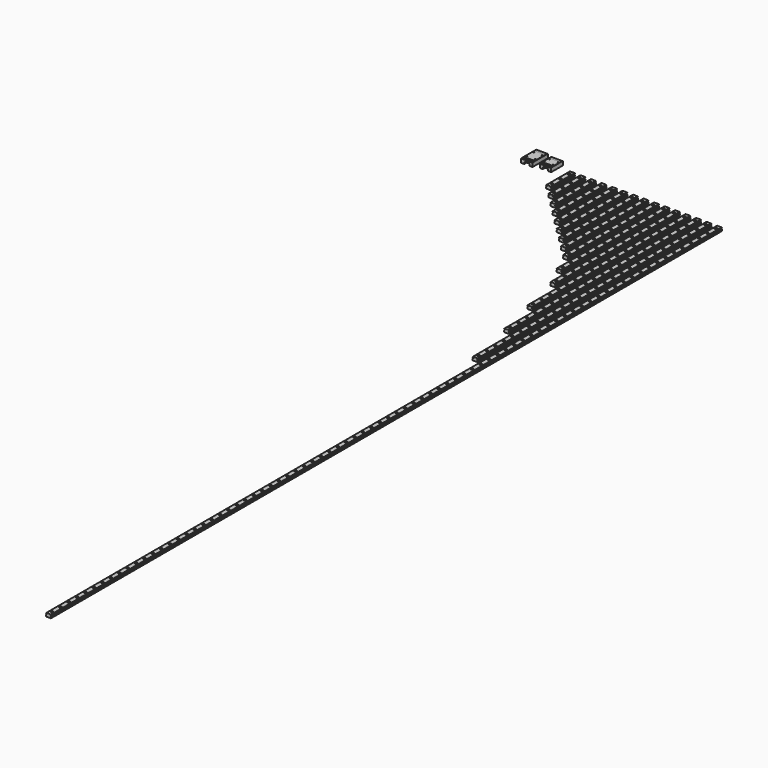
from build123d import *

# Parameters (mm, degrees)
F1_DEPTH           = 70
F2_DEPTH           = 95
F3_DEPTH           = 120
F4_DEPTH           = 145
F5_DEPTH           = 170
F6_DEPTH           = 195
F7_DEPTH           = 220
F8_DEPTH           = 245
F9_DEPTH           = 270
F10_DEPTH          = 320
F11_DEPTH          = 370
F12_DEPTH          = 470
F13_DEPTH          = 570
F14_DEPTH          = 695
F15_DEPTH          = 1995
F17_D              = 3.5
F17_CBORE_D        = 6
F17_CBORE_DEPTH    = 4.5
F17_2_D            = 3.5
F17_2_CBORE_D      = 6
F17_2_CBORE_DEPTH  = 4.5
F17_3_D            = 3.5
F17_3_CBORE_D      = 6
F17_3_CBORE_DEPTH  = 4.5
F17_4_D            = 3.5
F17_4_CBORE_D      = 6
F17_4_CBORE_DEPTH  = 4.5
F17_5_D            = 3.5
F17_5_CBORE_D      = 6
F17_5_CBORE_DEPTH  = 4.5
F17_6_D            = 3.5
F17_6_CBORE_D      = 6
F17_6_CBORE_DEPTH  = 4.5
F17_7_D            = 3.5
F17_7_CBORE_D      = 6
F17_7_CBORE_DEPTH  = 4.5
F17_8_D            = 3.5
F17_8_CBORE_D      = 6
F17_8_CBORE_DEPTH  = 4.5
F17_9_D            = 3.5
F17_9_CBORE_D      = 6
F17_9_CBORE_DEPTH  = 4.5
F17_10_D           = 3.5
F17_10_CBORE_D     = 6
F17_10_CBORE_DEPTH = 4.5
F18_D              = 3.5
F18_CBORE_D        = 6
F18_CBORE_DEPTH    = 4.5
F18_2_D            = 3.5
F18_2_CBORE_D      = 6
F18_2_CBORE_DEPTH  = 4.5
F18_3_D            = 3.5
F18_3_CBORE_D      = 6
F18_3_CBORE_DEPTH  = 4.5
F18_4_D            = 3.5
F18_4_CBORE_D      = 6
F18_4_CBORE_DEPTH  = 4.5
F19_D              = 3.5
F19_CBORE_D        = 6
F19_CBORE_DEPTH    = 4.5
F21_DEPTH          = 10.85
F23_DEPTH          = 6.5
F24_DEPTH          = 16.2
F26_DEPTH          = 6.5
F28_D              = 2.5
F28_DEPTH          = 5
F28_TIP            = 0.7510757738
F28_2_D            = 2.5
F28_2_DEPTH        = 5
F28_2_TIP          = 0.7510757738
F29_SIZE           = 0.49999
F29_2_SIZE         = 0.49999


# Not quite as in the source:
# - a fillet or chamfer is up to 0.001 mm smaller than in the source, because OpenCascade refuses the exact size


with BuildPart() as f1:
    # F0 (on Front) → F1 (new body)
    with BuildSketch(Plane.XZ):
        with BuildLine():
            Line((-5.5050252532, -4), (5.5050252532, -4))
            Line((5.5050252532, -4), (6, -3.5050252532))
            Line((6, -3.5050252532), (6, -0.0298848634))
            ThreePointArc((6, -0.0298848634), (5.4909752969, 0.2684521405), (5.150060681, 0.75))
            Line((5.150060681, 0.75), (4.45, 0.75))
            Line((4.45, 0.75), (4.45, 1.85))
            Line((4.45, 1.85), (5.150060681, 1.85))
            ThreePointArc((5.150060681, 1.85), (5.4909752969, 2.3315478595), (6, 2.6298848634))
            Line((6, 2.6298848634), (6, 3.5050252532))
            Line((6, 3.5050252532), (5.5050252532, 4))
            Line((5.5050252532, 4), (-5.5050252532, 4))
            Line((-5.5050252532, 4), (-6, 3.5050252532))
            Line((-6, 3.5050252532), (-6, 2.6298848634))
            ThreePointArc((-6, 2.6298848634), (-5.4909752969, 2.3315478595), (-5.150060681, 1.85))
            Line((-5.150060681, 1.85), (-4.45, 1.85))
            Line((-4.45, 1.85), (-4.45, 0.75))
            Line((-4.45, 0.75), (-5.150060681, 0.75))
            ThreePointArc((-5.150060681, 0.75), (-5.4909752969, 0.2684521405), (-6, -0.0298848634))
            Line((-6, -0.0298848634), (-6, -3.5050252532))
            Line((-6, -3.5050252532), (-5.5050252532, -4))
        make_face()
    extrude(amount=F1_DEPTH)

    # F17 (through all)
    with Locations(Plane.XY.offset(4)):
        with Locations((150, -10), (225, -35), (225, -10), (225, -60), (50, -60), (25, -10), (125, -60), (200, -10), (75, -10), (175, -35), (25, -60), (0, -35), (175, -10), (200, -35), (200, -60), (75, -60), (150, -60), (50, -35), (100, -10), (150, -35), (25, -35), (175, -60), (0, -10), (125, -35), (50, -10), (125, -10), (100, -35), (75, -35), (0, -60), (100, -60), (150, -85), (100, -85), (225, -85), (175, -85), (75, -85), (125, -85), (25, -85), (200, -85), (50, -85), (50, -110), (225, -110), (225, -135), (200, -110), (125, -110), (75, -110), (100, -135), (150, -135), (125, -135), (175, -135), (100, -110), (200, -135), (75, -135), (175, -110), (150, -110), (200, -160), (150, -160), (125, -160), (175, -160), (100, -160), (225, -160), (175, -185), (200, -185), (150, -185), (125, -185), (225, -185), (200, -260), (225, -310), (225, -260), (225, -285), (150, -210), (200, -235), (225, -210), (225, -235), (200, -210), (175, -235), (175, -210)):
            CounterBoreHole(F17_D / 2, F17_CBORE_D / 2, F17_CBORE_DEPTH)


with BuildPart() as f2:
    # F0 (on Front) → F2 (new body)
    with BuildSketch(Plane.XZ):
        with BuildLine():
            Line((19, -0.0298848634), (19, -3.5050252532))
            Line((19, -3.5050252532), (19.4949747468, -4))
            Line((19.4949747468, -4), (30.5050252532, -4))
            Line((30.5050252532, -4), (31, -3.5050252532))
            Line((31, -3.5050252532), (31, -0.0298848634))
            ThreePointArc((31, -0.0298848634), (30.4909752969, 0.2684521405), (30.150060681, 0.75))
            Line((30.150060681, 0.75), (29.45, 0.75))
            Line((29.45, 0.75), (29.45, 1.85))
            Line((29.45, 1.85), (30.150060681, 1.85))
            ThreePointArc((30.150060681, 1.85), (30.4909752969, 2.3315478595), (31, 2.6298848634))
            Line((31, 2.6298848634), (31, 3.5050252532))
            Line((31, 3.5050252532), (30.5050252532, 4))
            Line((30.5050252532, 4), (19.4949747468, 4))
            Line((19.4949747468, 4), (19, 3.5050252532))
            Line((19, 3.5050252532), (19, 2.6298848634))
            ThreePointArc((19, 2.6298848634), (19.5090247031, 2.3315478595), (19.849939319, 1.85))
            Line((19.849939319, 1.85), (20.55, 1.85))
            Line((20.55, 1.85), (20.55, 0.75))
            Line((20.55, 0.75), (19.849939319, 0.75))
            ThreePointArc((19.849939319, 0.75), (19.5090247031, 0.2684521405), (19, -0.0298848634))
        make_face()
    extrude(amount=F2_DEPTH)

    # F17#2 (through all)
    with Locations(Plane.XY.offset(4)):
        with Locations((150, -10), (225, -35), (225, -10), (225, -60), (50, -60), (25, -10), (125, -60), (200, -10), (75, -10), (175, -35), (25, -60), (0, -35), (175, -10), (200, -35), (200, -60), (75, -60), (150, -60), (50, -35), (100, -10), (150, -35), (25, -35), (175, -60), (0, -10), (125, -35), (50, -10), (125, -10), (100, -35), (75, -35), (0, -60), (100, -60), (150, -85), (100, -85), (225, -85), (175, -85), (75, -85), (125, -85), (25, -85), (200, -85), (50, -85), (50, -110), (225, -110), (225, -135), (200, -110), (125, -110), (75, -110), (100, -135), (150, -135), (125, -135), (175, -135), (100, -110), (200, -135), (75, -135), (175, -110), (150, -110), (200, -160), (150, -160), (125, -160), (175, -160), (100, -160), (225, -160), (175, -185), (200, -185), (150, -185), (125, -185), (225, -185), (200, -260), (225, -310), (225, -260), (225, -285), (150, -210), (200, -235), (225, -210), (225, -235), (200, -210), (175, -235), (175, -210)):
            CounterBoreHole(F17_2_D / 2, F17_2_CBORE_D / 2, F17_2_CBORE_DEPTH)


with BuildPart() as f3:
    # F0 (on Front) → F3 (new body)
    with BuildSketch(Plane.XZ):
        with BuildLine():
            Line((44, -0.0298848634), (44, -3.5050252532))
            Line((44, -3.5050252532), (44.4949747468, -4))
            Line((44.4949747468, -4), (55.5050252532, -4))
            Line((55.5050252532, -4), (56, -3.5050252532))
            Line((56, -3.5050252532), (56, -0.0298848634))
            ThreePointArc((56, -0.0298848634), (55.4909752969, 0.2684521405), (55.150060681, 0.75))
            Line((55.150060681, 0.75), (54.45, 0.75))
            Line((54.45, 0.75), (54.45, 1.85))
            Line((54.45, 1.85), (55.150060681, 1.85))
            ThreePointArc((55.150060681, 1.85), (55.4909752969, 2.3315478595), (56, 2.6298848634))
            Line((56, 2.6298848634), (56, 3.5050252532))
            Line((56, 3.5050252532), (55.5050252532, 4))
            Line((55.5050252532, 4), (44.4949747468, 4))
            Line((44.4949747468, 4), (44, 3.5050252532))
            Line((44, 3.5050252532), (44, 2.6298848634))
            ThreePointArc((44, 2.6298848634), (44.5090247031, 2.3315478595), (44.849939319, 1.85))
            Line((44.849939319, 1.85), (45.55, 1.85))
            Line((45.55, 1.85), (45.55, 0.75))
            Line((45.55, 0.75), (44.849939319, 0.75))
            ThreePointArc((44.849939319, 0.75), (44.5090247031, 0.2684521405), (44, -0.0298848634))
        make_face()
    extrude(amount=F3_DEPTH)

    # F17#3 (through all)
    with Locations(Plane.XY.offset(4)):
        with Locations((150, -10), (225, -35), (225, -10), (225, -60), (50, -60), (25, -10), (125, -60), (200, -10), (75, -10), (175, -35), (25, -60), (0, -35), (175, -10), (200, -35), (200, -60), (75, -60), (150, -60), (50, -35), (100, -10), (150, -35), (25, -35), (175, -60), (0, -10), (125, -35), (50, -10), (125, -10), (100, -35), (75, -35), (0, -60), (100, -60), (150, -85), (100, -85), (225, -85), (175, -85), (75, -85), (125, -85), (25, -85), (200, -85), (50, -85), (50, -110), (225, -110), (225, -135), (200, -110), (125, -110), (75, -110), (100, -135), (150, -135), (125, -135), (175, -135), (100, -110), (200, -135), (75, -135), (175, -110), (150, -110), (200, -160), (150, -160), (125, -160), (175, -160), (100, -160), (225, -160), (175, -185), (200, -185), (150, -185), (125, -185), (225, -185), (200, -260), (225, -310), (225, -260), (225, -285), (150, -210), (200, -235), (225, -210), (225, -235), (200, -210), (175, -235), (175, -210)):
            CounterBoreHole(F17_3_D / 2, F17_3_CBORE_D / 2, F17_3_CBORE_DEPTH)


with BuildPart() as f4:
    # F0 (on Front) → F4 (new body)
    with BuildSketch(Plane.XZ):
        with BuildLine():
            Line((69, -0.0298848634), (69, -3.5050252532))
            Line((69, -3.5050252532), (69.4949747468, -4))
            Line((69.4949747468, -4), (80.5050252532, -4))
            Line((80.5050252532, -4), (81, -3.5050252532))
            Line((81, -3.5050252532), (81, -0.0298848634))
            ThreePointArc((81, -0.0298848634), (80.4909752969, 0.2684521405), (80.150060681, 0.75))
            Line((80.150060681, 0.75), (79.45, 0.75))
            Line((79.45, 0.75), (79.45, 1.85))
            Line((79.45, 1.85), (80.150060681, 1.85))
            ThreePointArc((80.150060681, 1.85), (80.4909752969, 2.3315478595), (81, 2.6298848634))
            Line((81, 2.6298848634), (81, 3.5050252532))
            Line((81, 3.5050252532), (80.5050252532, 4))
            Line((80.5050252532, 4), (69.4949747468, 4))
            Line((69.4949747468, 4), (69, 3.5050252532))
            Line((69, 3.5050252532), (69, 2.6298848634))
            ThreePointArc((69, 2.6298848634), (69.5090247031, 2.3315478595), (69.849939319, 1.85))
            Line((69.849939319, 1.85), (70.55, 1.85))
            Line((70.55, 1.85), (70.55, 0.75))
            Line((70.55, 0.75), (69.849939319, 0.75))
            ThreePointArc((69.849939319, 0.75), (69.5090247031, 0.2684521405), (69, -0.0298848634))
        make_face()
    extrude(amount=F4_DEPTH)

    # F17#4 (through all)
    with Locations(Plane.XY.offset(4)):
        with Locations((150, -10), (225, -35), (225, -10), (225, -60), (50, -60), (25, -10), (125, -60), (200, -10), (75, -10), (175, -35), (25, -60), (0, -35), (175, -10), (200, -35), (200, -60), (75, -60), (150, -60), (50, -35), (100, -10), (150, -35), (25, -35), (175, -60), (0, -10), (125, -35), (50, -10), (125, -10), (100, -35), (75, -35), (0, -60), (100, -60), (150, -85), (100, -85), (225, -85), (175, -85), (75, -85), (125, -85), (25, -85), (200, -85), (50, -85), (50, -110), (225, -110), (225, -135), (200, -110), (125, -110), (75, -110), (100, -135), (150, -135), (125, -135), (175, -135), (100, -110), (200, -135), (75, -135), (175, -110), (150, -110), (200, -160), (150, -160), (125, -160), (175, -160), (100, -160), (225, -160), (175, -185), (200, -185), (150, -185), (125, -185), (225, -185), (200, -260), (225, -310), (225, -260), (225, -285), (150, -210), (200, -235), (225, -210), (225, -235), (200, -210), (175, -235), (175, -210)):
            CounterBoreHole(F17_4_D / 2, F17_4_CBORE_D / 2, F17_4_CBORE_DEPTH)


with BuildPart() as f5:
    # F0 (on Front) → F5 (new body)
    with BuildSketch(Plane.XZ):
        with BuildLine():
            Line((94, -0.0298848634), (94, -3.5050252532))
            Line((94, -3.5050252532), (94.4949747468, -4))
            Line((94.4949747468, -4), (105.5050252532, -4))
            Line((105.5050252532, -4), (106, -3.5050252532))
            Line((106, -3.5050252532), (106, -0.0298848634))
            ThreePointArc((106, -0.0298848634), (105.4909752969, 0.2684521405), (105.150060681, 0.75))
            Line((105.150060681, 0.75), (104.45, 0.75))
            Line((104.45, 0.75), (104.45, 1.85))
            Line((104.45, 1.85), (105.150060681, 1.85))
            ThreePointArc((105.150060681, 1.85), (105.4909752969, 2.3315478595), (106, 2.6298848634))
            Line((106, 2.6298848634), (106, 3.5050252532))
            Line((106, 3.5050252532), (105.5050252532, 4))
            Line((105.5050252532, 4), (94.4949747468, 4))
            Line((94.4949747468, 4), (94, 3.5050252532))
            Line((94, 3.5050252532), (94, 2.6298848634))
            ThreePointArc((94, 2.6298848634), (94.5090247031, 2.3315478595), (94.849939319, 1.85))
            Line((94.849939319, 1.85), (95.55, 1.85))
            Line((95.55, 1.85), (95.55, 0.75))
            Line((95.55, 0.75), (94.849939319, 0.75))
            ThreePointArc((94.849939319, 0.75), (94.5090247031, 0.2684521405), (94, -0.0298848634))
        make_face()
    extrude(amount=F5_DEPTH)

    # F17#5 (through all)
    with Locations(Plane.XY.offset(4)):
        with Locations((150, -10), (225, -35), (225, -10), (225, -60), (50, -60), (25, -10), (125, -60), (200, -10), (75, -10), (175, -35), (25, -60), (0, -35), (175, -10), (200, -35), (200, -60), (75, -60), (150, -60), (50, -35), (100, -10), (150, -35), (25, -35), (175, -60), (0, -10), (125, -35), (50, -10), (125, -10), (100, -35), (75, -35), (0, -60), (100, -60), (150, -85), (100, -85), (225, -85), (175, -85), (75, -85), (125, -85), (25, -85), (200, -85), (50, -85), (50, -110), (225, -110), (225, -135), (200, -110), (125, -110), (75, -110), (100, -135), (150, -135), (125, -135), (175, -135), (100, -110), (200, -135), (75, -135), (175, -110), (150, -110), (200, -160), (150, -160), (125, -160), (175, -160), (100, -160), (225, -160), (175, -185), (200, -185), (150, -185), (125, -185), (225, -185), (200, -260), (225, -310), (225, -260), (225, -285), (150, -210), (200, -235), (225, -210), (225, -235), (200, -210), (175, -235), (175, -210)):
            CounterBoreHole(F17_5_D / 2, F17_5_CBORE_D / 2, F17_5_CBORE_DEPTH)


with BuildPart() as f6:
    # F0 (on Front) → F6 (new body)
    with BuildSketch(Plane.XZ):
        with BuildLine():
            Line((119, -0.0298848634), (119, -3.5050252532))
            Line((119, -3.5050252532), (119.4949747468, -4))
            Line((119.4949747468, -4), (130.5050252532, -4))
            Line((130.5050252532, -4), (131, -3.5050252532))
            Line((131, -3.5050252532), (131, -0.0298848634))
            ThreePointArc((131, -0.0298848634), (130.4909752969, 0.2684521405), (130.150060681, 0.75))
            Line((130.150060681, 0.75), (129.45, 0.75))
            Line((129.45, 0.75), (129.45, 1.85))
            Line((129.45, 1.85), (130.150060681, 1.85))
            ThreePointArc((130.150060681, 1.85), (130.4909752969, 2.3315478595), (131, 2.6298848634))
            Line((131, 2.6298848634), (131, 3.5050252532))
            Line((131, 3.5050252532), (130.5050252532, 4))
            Line((130.5050252532, 4), (119.4949747468, 4))
            Line((119.4949747468, 4), (119, 3.5050252532))
            Line((119, 3.5050252532), (119, 2.6298848634))
            ThreePointArc((119, 2.6298848634), (119.5090247031, 2.3315478595), (119.849939319, 1.85))
            Line((119.849939319, 1.85), (120.55, 1.85))
            Line((120.55, 1.85), (120.55, 0.75))
            Line((120.55, 0.75), (119.849939319, 0.75))
            ThreePointArc((119.849939319, 0.75), (119.5090247031, 0.2684521405), (119, -0.0298848634))
        make_face()
    extrude(amount=F6_DEPTH)

    # F17#6 (through all)
    with Locations(Plane.XY.offset(4)):
        with Locations((150, -10), (225, -35), (225, -10), (225, -60), (50, -60), (25, -10), (125, -60), (200, -10), (75, -10), (175, -35), (25, -60), (0, -35), (175, -10), (200, -35), (200, -60), (75, -60), (150, -60), (50, -35), (100, -10), (150, -35), (25, -35), (175, -60), (0, -10), (125, -35), (50, -10), (125, -10), (100, -35), (75, -35), (0, -60), (100, -60), (150, -85), (100, -85), (225, -85), (175, -85), (75, -85), (125, -85), (25, -85), (200, -85), (50, -85), (50, -110), (225, -110), (225, -135), (200, -110), (125, -110), (75, -110), (100, -135), (150, -135), (125, -135), (175, -135), (100, -110), (200, -135), (75, -135), (175, -110), (150, -110), (200, -160), (150, -160), (125, -160), (175, -160), (100, -160), (225, -160), (175, -185), (200, -185), (150, -185), (125, -185), (225, -185), (200, -260), (225, -310), (225, -260), (225, -285), (150, -210), (200, -235), (225, -210), (225, -235), (200, -210), (175, -235), (175, -210)):
            CounterBoreHole(F17_6_D / 2, F17_6_CBORE_D / 2, F17_6_CBORE_DEPTH)


with BuildPart() as f7:
    # F0 (on Front) → F7 (new body)
    with BuildSketch(Plane.XZ):
        with BuildLine():
            Line((144, -0.0298848634), (144, -3.5050252532))
            Line((144, -3.5050252532), (144.4949747468, -4))
            Line((144.4949747468, -4), (155.5050252532, -4))
            Line((155.5050252532, -4), (156, -3.5050252532))
            Line((156, -3.5050252532), (156, -0.0298848634))
            ThreePointArc((156, -0.0298848634), (155.4909752969, 0.2684521405), (155.150060681, 0.75))
            Line((155.150060681, 0.75), (154.45, 0.75))
            Line((154.45, 0.75), (154.45, 1.85))
            Line((154.45, 1.85), (155.150060681, 1.85))
            ThreePointArc((155.150060681, 1.85), (155.4909752969, 2.3315478595), (156, 2.6298848634))
            Line((156, 2.6298848634), (156, 3.5050252532))
            Line((156, 3.5050252532), (155.5050252532, 4))
            Line((155.5050252532, 4), (144.4949747468, 4))
            Line((144.4949747468, 4), (144, 3.5050252532))
            Line((144, 3.5050252532), (144, 2.6298848634))
            ThreePointArc((144, 2.6298848634), (144.5090247031, 2.3315478595), (144.849939319, 1.85))
            Line((144.849939319, 1.85), (145.55, 1.85))
            Line((145.55, 1.85), (145.55, 0.75))
            Line((145.55, 0.75), (144.849939319, 0.75))
            ThreePointArc((144.849939319, 0.75), (144.5090247031, 0.2684521405), (144, -0.0298848634))
        make_face()
    extrude(amount=F7_DEPTH)

    # F17#7 (through all)
    with Locations(Plane.XY.offset(4)):
        with Locations((150, -10), (225, -35), (225, -10), (225, -60), (50, -60), (25, -10), (125, -60), (200, -10), (75, -10), (175, -35), (25, -60), (0, -35), (175, -10), (200, -35), (200, -60), (75, -60), (150, -60), (50, -35), (100, -10), (150, -35), (25, -35), (175, -60), (0, -10), (125, -35), (50, -10), (125, -10), (100, -35), (75, -35), (0, -60), (100, -60), (150, -85), (100, -85), (225, -85), (175, -85), (75, -85), (125, -85), (25, -85), (200, -85), (50, -85), (50, -110), (225, -110), (225, -135), (200, -110), (125, -110), (75, -110), (100, -135), (150, -135), (125, -135), (175, -135), (100, -110), (200, -135), (75, -135), (175, -110), (150, -110), (200, -160), (150, -160), (125, -160), (175, -160), (100, -160), (225, -160), (175, -185), (200, -185), (150, -185), (125, -185), (225, -185), (200, -260), (225, -310), (225, -260), (225, -285), (150, -210), (200, -235), (225, -210), (225, -235), (200, -210), (175, -235), (175, -210)):
            CounterBoreHole(F17_7_D / 2, F17_7_CBORE_D / 2, F17_7_CBORE_DEPTH)


with BuildPart() as f8:
    # F0 (on Front) → F8 (new body)
    with BuildSketch(Plane.XZ):
        with BuildLine():
            Line((169, -0.0298848634), (169, -3.5050252532))
            Line((169, -3.5050252532), (169.4949747468, -4))
            Line((169.4949747468, -4), (180.5050252532, -4))
            Line((180.5050252532, -4), (181, -3.5050252532))
            Line((181, -3.5050252532), (181, -0.0298848634))
            ThreePointArc((181, -0.0298848634), (180.4909752969, 0.2684521405), (180.150060681, 0.75))
            Line((180.150060681, 0.75), (179.45, 0.75))
            Line((179.45, 0.75), (179.45, 1.85))
            Line((179.45, 1.85), (180.150060681, 1.85))
            ThreePointArc((180.150060681, 1.85), (180.4909752969, 2.3315478595), (181, 2.6298848634))
            Line((181, 2.6298848634), (181, 3.5050252532))
            Line((181, 3.5050252532), (180.5050252532, 4))
            Line((180.5050252532, 4), (169.4949747468, 4))
            Line((169.4949747468, 4), (169, 3.5050252532))
            Line((169, 3.5050252532), (169, 2.6298848634))
            ThreePointArc((169, 2.6298848634), (169.5090247031, 2.3315478595), (169.849939319, 1.85))
            Line((169.849939319, 1.85), (170.55, 1.85))
            Line((170.55, 1.85), (170.55, 0.75))
            Line((170.55, 0.75), (169.849939319, 0.75))
            ThreePointArc((169.849939319, 0.75), (169.5090247031, 0.2684521405), (169, -0.0298848634))
        make_face()
    extrude(amount=F8_DEPTH)

    # F17#8 (through all)
    with Locations(Plane.XY.offset(4)):
        with Locations((150, -10), (225, -35), (225, -10), (225, -60), (50, -60), (25, -10), (125, -60), (200, -10), (75, -10), (175, -35), (25, -60), (0, -35), (175, -10), (200, -35), (200, -60), (75, -60), (150, -60), (50, -35), (100, -10), (150, -35), (25, -35), (175, -60), (0, -10), (125, -35), (50, -10), (125, -10), (100, -35), (75, -35), (0, -60), (100, -60), (150, -85), (100, -85), (225, -85), (175, -85), (75, -85), (125, -85), (25, -85), (200, -85), (50, -85), (50, -110), (225, -110), (225, -135), (200, -110), (125, -110), (75, -110), (100, -135), (150, -135), (125, -135), (175, -135), (100, -110), (200, -135), (75, -135), (175, -110), (150, -110), (200, -160), (150, -160), (125, -160), (175, -160), (100, -160), (225, -160), (175, -185), (200, -185), (150, -185), (125, -185), (225, -185), (200, -260), (225, -310), (225, -260), (225, -285), (150, -210), (200, -235), (225, -210), (225, -235), (200, -210), (175, -235), (175, -210)):
            CounterBoreHole(F17_8_D / 2, F17_8_CBORE_D / 2, F17_8_CBORE_DEPTH)


with BuildPart() as f9:
    # F0 (on Front) → F9 (new body)
    with BuildSketch(Plane.XZ):
        with BuildLine():
            Line((194, -0.0298848634), (194, -3.5050252532))
            Line((194, -3.5050252532), (194.4949747468, -4))
            Line((194.4949747468, -4), (205.5050252532, -4))
            Line((205.5050252532, -4), (206, -3.5050252532))
            Line((206, -3.5050252532), (206, -0.0298848634))
            ThreePointArc((206, -0.0298848634), (205.4909752969, 0.2684521405), (205.150060681, 0.75))
            Line((205.150060681, 0.75), (204.45, 0.75))
            Line((204.45, 0.75), (204.45, 1.85))
            Line((204.45, 1.85), (205.150060681, 1.85))
            ThreePointArc((205.150060681, 1.85), (205.4909752969, 2.3315478595), (206, 2.6298848634))
            Line((206, 2.6298848634), (206, 3.5050252532))
            Line((206, 3.5050252532), (205.5050252532, 4))
            Line((205.5050252532, 4), (194.4949747468, 4))
            Line((194.4949747468, 4), (194, 3.5050252532))
            Line((194, 3.5050252532), (194, 2.6298848634))
            ThreePointArc((194, 2.6298848634), (194.5090247031, 2.3315478595), (194.849939319, 1.85))
            Line((194.849939319, 1.85), (195.55, 1.85))
            Line((195.55, 1.85), (195.55, 0.75))
            Line((195.55, 0.75), (194.849939319, 0.75))
            ThreePointArc((194.849939319, 0.75), (194.5090247031, 0.2684521405), (194, -0.0298848634))
        make_face()
    extrude(amount=F9_DEPTH)

    # F17#9 (through all)
    with Locations(Plane.XY.offset(4)):
        with Locations((150, -10), (225, -35), (225, -10), (225, -60), (50, -60), (25, -10), (125, -60), (200, -10), (75, -10), (175, -35), (25, -60), (0, -35), (175, -10), (200, -35), (200, -60), (75, -60), (150, -60), (50, -35), (100, -10), (150, -35), (25, -35), (175, -60), (0, -10), (125, -35), (50, -10), (125, -10), (100, -35), (75, -35), (0, -60), (100, -60), (150, -85), (100, -85), (225, -85), (175, -85), (75, -85), (125, -85), (25, -85), (200, -85), (50, -85), (50, -110), (225, -110), (225, -135), (200, -110), (125, -110), (75, -110), (100, -135), (150, -135), (125, -135), (175, -135), (100, -110), (200, -135), (75, -135), (175, -110), (150, -110), (200, -160), (150, -160), (125, -160), (175, -160), (100, -160), (225, -160), (175, -185), (200, -185), (150, -185), (125, -185), (225, -185), (200, -260), (225, -310), (225, -260), (225, -285), (150, -210), (200, -235), (225, -210), (225, -235), (200, -210), (175, -235), (175, -210)):
            CounterBoreHole(F17_9_D / 2, F17_9_CBORE_D / 2, F17_9_CBORE_DEPTH)


with BuildPart() as f10:
    # F0 (on Front) → F10 (new body)
    with BuildSketch(Plane.XZ):
        with BuildLine():
            Line((219, -0.0298848634), (219, -3.5050252532))
            Line((219, -3.5050252532), (219.4949747468, -4))
            Line((219.4949747468, -4), (230.5050252532, -4))
            Line((230.5050252532, -4), (231, -3.5050252532))
            Line((231, -3.5050252532), (231, -0.0298848634))
            ThreePointArc((231, -0.0298848634), (230.4909752969, 0.2684521405), (230.150060681, 0.75))
            Line((230.150060681, 0.75), (229.45, 0.75))
            Line((229.45, 0.75), (229.45, 1.85))
            Line((229.45, 1.85), (230.150060681, 1.85))
            ThreePointArc((230.150060681, 1.85), (230.4909752969, 2.3315478595), (231, 2.6298848634))
            Line((231, 2.6298848634), (231, 3.5050252532))
            Line((231, 3.5050252532), (230.5050252532, 4))
            Line((230.5050252532, 4), (219.4949747468, 4))
            Line((219.4949747468, 4), (219, 3.5050252532))
            Line((219, 3.5050252532), (219, 2.6298848634))
            ThreePointArc((219, 2.6298848634), (219.5090247031, 2.3315478595), (219.849939319, 1.85))
            Line((219.849939319, 1.85), (220.55, 1.85))
            Line((220.55, 1.85), (220.55, 0.75))
            Line((220.55, 0.75), (219.849939319, 0.75))
            ThreePointArc((219.849939319, 0.75), (219.5090247031, 0.2684521405), (219, -0.0298848634))
        make_face()
    extrude(amount=F10_DEPTH)

    # F17#10 (through all)
    with Locations(Plane.XY.offset(4)):
        with Locations((150, -10), (225, -35), (225, -10), (225, -60), (50, -60), (25, -10), (125, -60), (200, -10), (75, -10), (175, -35), (25, -60), (0, -35), (175, -10), (200, -35), (200, -60), (75, -60), (150, -60), (50, -35), (100, -10), (150, -35), (25, -35), (175, -60), (0, -10), (125, -35), (50, -10), (125, -10), (100, -35), (75, -35), (0, -60), (100, -60), (150, -85), (100, -85), (225, -85), (175, -85), (75, -85), (125, -85), (25, -85), (200, -85), (50, -85), (50, -110), (225, -110), (225, -135), (200, -110), (125, -110), (75, -110), (100, -135), (150, -135), (125, -135), (175, -135), (100, -110), (200, -135), (75, -135), (175, -110), (150, -110), (200, -160), (150, -160), (125, -160), (175, -160), (100, -160), (225, -160), (175, -185), (200, -185), (150, -185), (125, -185), (225, -185), (200, -260), (225, -310), (225, -260), (225, -285), (150, -210), (200, -235), (225, -210), (225, -235), (200, -210), (175, -235), (175, -210)):
            CounterBoreHole(F17_10_D / 2, F17_10_CBORE_D / 2, F17_10_CBORE_DEPTH)


with BuildPart() as f11:
    # F0 (on Front) → F11 (new body)
    with BuildSketch(Plane.XZ):
        with BuildLine():
            Line((244, -0.0298848634), (244, -3.5050252532))
            Line((244, -3.5050252532), (244.4949747468, -4))
            Line((244.4949747468, -4), (255.5050252532, -4))
            Line((255.5050252532, -4), (256, -3.5050252532))
            Line((256, -3.5050252532), (256, -0.0298848634))
            ThreePointArc((256, -0.0298848634), (255.4909752969, 0.2684521405), (255.150060681, 0.75))
            Line((255.150060681, 0.75), (254.45, 0.75))
            Line((254.45, 0.75), (254.45, 1.85))
            Line((254.45, 1.85), (255.150060681, 1.85))
            ThreePointArc((255.150060681, 1.85), (255.4909752969, 2.3315478595), (256, 2.6298848634))
            Line((256, 2.6298848634), (256, 3.5050252532))
            Line((256, 3.5050252532), (255.5050252532, 4))
            Line((255.5050252532, 4), (244.4949747468, 4))
            Line((244.4949747468, 4), (244, 3.5050252532))
            Line((244, 3.5050252532), (244, 2.6298848634))
            ThreePointArc((244, 2.6298848634), (244.5090247031, 2.3315478595), (244.849939319, 1.85))
            Line((244.849939319, 1.85), (245.55, 1.85))
            Line((245.55, 1.85), (245.55, 0.75))
            Line((245.55, 0.75), (244.849939319, 0.75))
            ThreePointArc((244.849939319, 0.75), (244.5090247031, 0.2684521405), (244, -0.0298848634))
        make_face()
    extrude(amount=F11_DEPTH)

    # F18 (through all)
    with Locations(Plane.XY.offset(4)):
        with Locations((250, -85), (250, -110), (250, -210), (250, -185), (250, -260), (250, -310), (250, -135), (250, -35), (250, -285), (250, -360), (250, -60), (250, -160), (250, -10), (250, -235), (250, -335), (275, -460), (275, -60), (275, -285), (275, -10), (275, -410), (275, -210), (275, -35), (275, -435), (275, -335), (275, -235), (275, -135), (275, -310), (275, -110), (275, -385), (275, -185), (275, -160), (275, -85), (275, -360), (275, -260), (300, -410), (300, -310), (300, -535), (300, -510), (300, -235), (300, -335), (300, -260), (300, -385), (300, -110), (300, -35), (300, -210), (300, -485), (300, -85), (300, -185), (300, -460), (300, -560), (300, -60), (300, -160), (300, -435), (300, -360), (300, -10), (300, -135), (300, -285), (325, -60), (325, -635), (325, -410), (325, -535), (325, -335), (325, -260), (325, -560), (325, -385), (325, -660), (325, -110), (325, -10), (325, -435), (325, -135), (325, -160), (325, -35), (325, -185), (325, -460), (325, -510), (325, -310), (325, -285), (325, -235), (325, -585), (325, -610), (325, -360), (325, -685), (325, -85), (325, -485), (325, -210)):
            CounterBoreHole(F18_D / 2, F18_CBORE_D / 2, F18_CBORE_DEPTH)


with BuildPart() as f12:
    # F0 (on Front) → F12 (new body)
    with BuildSketch(Plane.XZ):
        with BuildLine():
            Line((269, -0.0298848634), (269, -3.5050252532))
            Line((269, -3.5050252532), (269.4949747468, -4))
            Line((269.4949747468, -4), (280.5050252532, -4))
            Line((280.5050252532, -4), (281, -3.5050252532))
            Line((281, -3.5050252532), (281, -0.0298848634))
            ThreePointArc((281, -0.0298848634), (280.4909752969, 0.2684521405), (280.150060681, 0.75))
            Line((280.150060681, 0.75), (279.45, 0.75))
            Line((279.45, 0.75), (279.45, 1.85))
            Line((279.45, 1.85), (280.150060681, 1.85))
            ThreePointArc((280.150060681, 1.85), (280.4909752969, 2.3315478595), (281, 2.6298848634))
            Line((281, 2.6298848634), (281, 3.5050252532))
            Line((281, 3.5050252532), (280.5050252532, 4))
            Line((280.5050252532, 4), (269.4949747468, 4))
            Line((269.4949747468, 4), (269, 3.5050252532))
            Line((269, 3.5050252532), (269, 2.6298848634))
            ThreePointArc((269, 2.6298848634), (269.5090247031, 2.3315478595), (269.849939319, 1.85))
            Line((269.849939319, 1.85), (270.55, 1.85))
            Line((270.55, 1.85), (270.55, 0.75))
            Line((270.55, 0.75), (269.849939319, 0.75))
            ThreePointArc((269.849939319, 0.75), (269.5090247031, 0.2684521405), (269, -0.0298848634))
        make_face()
    extrude(amount=F12_DEPTH)

    # F18#2 (through all)
    with Locations(Plane.XY.offset(4)):
        with Locations((250, -85), (250, -110), (250, -210), (250, -185), (250, -260), (250, -310), (250, -135), (250, -35), (250, -285), (250, -360), (250, -60), (250, -160), (250, -10), (250, -235), (250, -335), (275, -460), (275, -60), (275, -285), (275, -10), (275, -410), (275, -210), (275, -35), (275, -435), (275, -335), (275, -235), (275, -135), (275, -310), (275, -110), (275, -385), (275, -185), (275, -160), (275, -85), (275, -360), (275, -260), (300, -410), (300, -310), (300, -535), (300, -510), (300, -235), (300, -335), (300, -260), (300, -385), (300, -110), (300, -35), (300, -210), (300, -485), (300, -85), (300, -185), (300, -460), (300, -560), (300, -60), (300, -160), (300, -435), (300, -360), (300, -10), (300, -135), (300, -285), (325, -60), (325, -635), (325, -410), (325, -535), (325, -335), (325, -260), (325, -560), (325, -385), (325, -660), (325, -110), (325, -10), (325, -435), (325, -135), (325, -160), (325, -35), (325, -185), (325, -460), (325, -510), (325, -310), (325, -285), (325, -235), (325, -585), (325, -610), (325, -360), (325, -685), (325, -85), (325, -485), (325, -210)):
            CounterBoreHole(F18_2_D / 2, F18_2_CBORE_D / 2, F18_2_CBORE_DEPTH)


with BuildPart() as f13:
    # F0 (on Front) → F13 (new body)
    with BuildSketch(Plane.XZ):
        with BuildLine():
            Line((294, -0.0298848634), (294, -3.5050252532))
            Line((294, -3.5050252532), (294.4949747468, -4))
            Line((294.4949747468, -4), (305.5050252532, -4))
            Line((305.5050252532, -4), (306, -3.5050252532))
            Line((306, -3.5050252532), (306, -0.0298848634))
            ThreePointArc((306, -0.0298848634), (305.4909752969, 0.2684521405), (305.150060681, 0.75))
            Line((305.150060681, 0.75), (304.45, 0.75))
            Line((304.45, 0.75), (304.45, 1.85))
            Line((304.45, 1.85), (305.150060681, 1.85))
            ThreePointArc((305.150060681, 1.85), (305.4909752969, 2.3315478595), (306, 2.6298848634))
            Line((306, 2.6298848634), (306, 3.5050252532))
            Line((306, 3.5050252532), (305.5050252532, 4))
            Line((305.5050252532, 4), (294.4949747468, 4))
            Line((294.4949747468, 4), (294, 3.5050252532))
            Line((294, 3.5050252532), (294, 2.6298848634))
            ThreePointArc((294, 2.6298848634), (294.5090247031, 2.3315478595), (294.849939319, 1.85))
            Line((294.849939319, 1.85), (295.55, 1.85))
            Line((295.55, 1.85), (295.55, 0.75))
            Line((295.55, 0.75), (294.849939319, 0.75))
            ThreePointArc((294.849939319, 0.75), (294.5090247031, 0.2684521405), (294, -0.0298848634))
        make_face()
    extrude(amount=F13_DEPTH)

    # F18#3 (through all)
    with Locations(Plane.XY.offset(4)):
        with Locations((250, -85), (250, -110), (250, -210), (250, -185), (250, -260), (250, -310), (250, -135), (250, -35), (250, -285), (250, -360), (250, -60), (250, -160), (250, -10), (250, -235), (250, -335), (275, -460), (275, -60), (275, -285), (275, -10), (275, -410), (275, -210), (275, -35), (275, -435), (275, -335), (275, -235), (275, -135), (275, -310), (275, -110), (275, -385), (275, -185), (275, -160), (275, -85), (275, -360), (275, -260), (300, -410), (300, -310), (300, -535), (300, -510), (300, -235), (300, -335), (300, -260), (300, -385), (300, -110), (300, -35), (300, -210), (300, -485), (300, -85), (300, -185), (300, -460), (300, -560), (300, -60), (300, -160), (300, -435), (300, -360), (300, -10), (300, -135), (300, -285), (325, -60), (325, -635), (325, -410), (325, -535), (325, -335), (325, -260), (325, -560), (325, -385), (325, -660), (325, -110), (325, -10), (325, -435), (325, -135), (325, -160), (325, -35), (325, -185), (325, -460), (325, -510), (325, -310), (325, -285), (325, -235), (325, -585), (325, -610), (325, -360), (325, -685), (325, -85), (325, -485), (325, -210)):
            CounterBoreHole(F18_3_D / 2, F18_3_CBORE_D / 2, F18_3_CBORE_DEPTH)


with BuildPart() as f14:
    # F0 (on Front) → F14 (new body)
    with BuildSketch(Plane.XZ):
        with BuildLine():
            Line((319, -0.0298848634), (319, -3.5050252532))
            Line((319, -3.5050252532), (319.4949747468, -4))
            Line((319.4949747468, -4), (330.5050252532, -4))
            Line((330.5050252532, -4), (331, -3.5050252532))
            Line((331, -3.5050252532), (331, -0.0298848634))
            ThreePointArc((331, -0.0298848634), (330.4909752969, 0.2684521405), (330.150060681, 0.75))
            Line((330.150060681, 0.75), (329.45, 0.75))
            Line((329.45, 0.75), (329.45, 1.85))
            Line((329.45, 1.85), (330.150060681, 1.85))
            ThreePointArc((330.150060681, 1.85), (330.4909752969, 2.3315478595), (331, 2.6298848634))
            Line((331, 2.6298848634), (331, 3.5050252532))
            Line((331, 3.5050252532), (330.5050252532, 4))
            Line((330.5050252532, 4), (319.4949747468, 4))
            Line((319.4949747468, 4), (319, 3.5050252532))
            Line((319, 3.5050252532), (319, 2.6298848634))
            ThreePointArc((319, 2.6298848634), (319.5090247031, 2.3315478595), (319.849939319, 1.85))
            Line((319.849939319, 1.85), (320.55, 1.85))
            Line((320.55, 1.85), (320.55, 0.75))
            Line((320.55, 0.75), (319.849939319, 0.75))
            ThreePointArc((319.849939319, 0.75), (319.5090247031, 0.2684521405), (319, -0.0298848634))
        make_face()
    extrude(amount=F14_DEPTH)

    # F18#4 (through all)
    with Locations(Plane.XY.offset(4)):
        with Locations((250, -85), (250, -110), (250, -210), (250, -185), (250, -260), (250, -310), (250, -135), (250, -35), (250, -285), (250, -360), (250, -60), (250, -160), (250, -10), (250, -235), (250, -335), (275, -460), (275, -60), (275, -285), (275, -10), (275, -410), (275, -210), (275, -35), (275, -435), (275, -335), (275, -235), (275, -135), (275, -310), (275, -110), (275, -385), (275, -185), (275, -160), (275, -85), (275, -360), (275, -260), (300, -410), (300, -310), (300, -535), (300, -510), (300, -235), (300, -335), (300, -260), (300, -385), (300, -110), (300, -35), (300, -210), (300, -485), (300, -85), (300, -185), (300, -460), (300, -560), (300, -60), (300, -160), (300, -435), (300, -360), (300, -10), (300, -135), (300, -285), (325, -60), (325, -635), (325, -410), (325, -535), (325, -335), (325, -260), (325, -560), (325, -385), (325, -660), (325, -110), (325, -10), (325, -435), (325, -135), (325, -160), (325, -35), (325, -185), (325, -460), (325, -510), (325, -310), (325, -285), (325, -235), (325, -585), (325, -610), (325, -360), (325, -685), (325, -85), (325, -485), (325, -210)):
            CounterBoreHole(F18_4_D / 2, F18_4_CBORE_D / 2, F18_4_CBORE_DEPTH)


with BuildPart() as f15:
    # F0 (on Front) → F15 (new body)
    with BuildSketch(Plane.XZ):
        with BuildLine():
            Line((344, -0.0298848634), (344, -3.5050252532))
            Line((344, -3.5050252532), (344.4949747468, -4))
            Line((344.4949747468, -4), (355.5050252532, -4))
            Line((355.5050252532, -4), (356, -3.5050252532))
            Line((356, -3.5050252532), (356, -0.0298848634))
            ThreePointArc((356, -0.0298848634), (355.4909752969, 0.2684521405), (355.150060681, 0.75))
            Line((355.150060681, 0.75), (354.45, 0.75))
            Line((354.45, 0.75), (354.45, 1.85))
            Line((354.45, 1.85), (355.150060681, 1.85))
            ThreePointArc((355.150060681, 1.85), (355.4909752969, 2.3315478595), (356, 2.6298848634))
            Line((356, 2.6298848634), (356, 3.5050252532))
            Line((356, 3.5050252532), (355.5050252532, 4))
            Line((355.5050252532, 4), (344.4949747468, 4))
            Line((344.4949747468, 4), (344, 3.5050252532))
            Line((344, 3.5050252532), (344, 2.6298848634))
            ThreePointArc((344, 2.6298848634), (344.5090247031, 2.3315478595), (344.849939319, 1.85))
            Line((344.849939319, 1.85), (345.55, 1.85))
            Line((345.55, 1.85), (345.55, 0.75))
            Line((345.55, 0.75), (344.849939319, 0.75))
            ThreePointArc((344.849939319, 0.75), (344.5090247031, 0.2684521405), (344, -0.0298848634))
        make_face()
    extrude(amount=F15_DEPTH)

    # F19 (through all)
    with Locations(Plane.XY.offset(4)):
        with Locations((350, -310), (350, -160), (350, -110), (350, -260), (350, -335), (350, -210), (350, -460), (350, -10), (350, -635), (350, -560), (350, -235), (350, -610), (350, -435), (350, -410), (350, -735), (350, -660), (350, -360), (350, -35), (350, -135), (350, -385), (350, -485), (350, -85), (350, -185), (350, -285), (350, -535), (350, -510), (350, -685), (350, -585), (350, -60), (350, -710), (350, -1335), (350, -810), (350, -910), (350, -1460), (350, -1360), (350, -935), (350, -1435), (350, -1310), (350, -760), (350, -1510), (350, -1010), (350, -1135), (350, -1110), (350, -1260), (350, -1235), (350, -1385), (350, -960), (350, -1185), (350, -1585), (350, -860), (350, -1410), (350, -835), (350, -1160), (350, -1210), (350, -1535), (350, -1085), (350, -1060), (350, -885), (350, -1485), (350, -785), (350, -1285), (350, -1560), (350, -1035), (350, -985), (350, -1610), (350, -1935), (350, -1710), (350, -1860), (350, -1660), (350, -1985), (350, -1635), (350, -1810), (350, -1960), (350, -1760), (350, -1910), (350, -1785), (350, -1735), (350, -1835), (350, -1885), (350, -1685)):
            CounterBoreHole(F19_D / 2, F19_CBORE_D / 2, F19_CBORE_DEPTH)


with BuildPart() as f21:
    # F20 (on Front) → F21 (new body)
    with BuildSketch(Plane.XZ):
        with BuildLine():
            Line((-36.5, 8.5), (-63.5, 8.5))
            Line((-63.5, 8.5), (-63.5, -1))
            Line((-63.5, -1), (-56, -1))
            Line((-56, -1), (-56, -0.1))
            ThreePointArc((-56, -0.1), (-57.4, 1.3), (-56, 2.7))
            Line((-56, 2.7), (-56, 4))
            Line((-56, 4), (-50, 4))
            Line((-50, 4), (-44, 4))
            Line((-44, 4), (-44, 2.7))
            ThreePointArc((-44, 2.7), (-42.6, 1.3), (-44, -0.1))
            Line((-44, -0.1), (-44, -1))
            Line((-44, -1), (-36.5, -1))
            Line((-36.5, -1), (-36.5, 8.5))
        make_face()
        Polygon((-36.5, 9), (-50, 9), (-63.5, 9), (-63.5, 8.5), (-36.5, 8.5), align=None)
    extrude(amount=F21_DEPTH)

    # F22 (on face) → F23 (join)
    with BuildSketch(Plane.XZ.offset(10.85)):
        with BuildLine():
            Line((-36.5, 8.5), (-63.5, 8.5))
            Line((-63.5, 8.5), (-63.5, -1))
            Line((-63.5, -1), (-56, -1))
            Line((-56, -1), (-56, -0.1))
            ThreePointArc((-56, -0.1), (-57.4, 1.3), (-56, 2.7))
            Line((-56, 2.7), (-56, 4))
            Line((-56, 4), (-44, 4))
            Line((-44, 4), (-44, 2.7))
            ThreePointArc((-44, 2.7), (-42.6, 1.3), (-44, -0.1))
            Line((-44, -0.1), (-44, -1))
            Line((-44, -1), (-36.5, -1))
            Line((-36.5, -1), (-36.5, 8.5))
        make_face()
        with BuildLine():
            ThreePointArc((-56, 2.7), (-57.4, 1.3), (-56, -0.1))
            Line((-56, -0.1), (-56, 2.7))
        make_face()
        with BuildLine():
            Line((-44, 2.7), (-44, -0.1))
            ThreePointArc((-44, -0.1), (-42.6, 1.3), (-44, 2.7))
        make_face()
    extrude(amount=F23_DEPTH)

    # F28
    with Locations(Plane.XY.offset(9)):
        with Locations((-100, -10), (-80, -10), (-60, -7.5), (-40, -7.5)):
            Hole(F28_D / 2, depth=F28_DEPTH)
            with Locations((0, 0, -(F28_DEPTH + F28_TIP / 2))):  # 118° drill point
                Cone(0, F28_D / 2, F28_TIP, mode=Mode.SUBTRACT)

    # F29#2 (size 0.5 in the source; OpenCascade refuses exactly that, so slightly less here)
    f29_2_edges = [f21.edges().sort_by_distance(p)[0] for p in [
        (-50, -17.35, 8.5),
        (-50, -10.85, 9),
        (-63.5, -5.425, 9),
        (-36.5, -5.425, 9),
    ]]
    chamfer(f29_2_edges, length=F29_2_SIZE)



with BuildPart() as f24:
    # F20 (on Front) → F24 (new body)
    with BuildSketch(Plane.XZ):
        with BuildLine():
            ThreePointArc((-96, -0.1), (-97.4, 1.3), (-96, 2.7))
            Line((-96, 2.7), (-96, 4))
            Line((-96, 4), (-90, 4))
            Line((-90, 4), (-84, 4))
            Line((-84, 4), (-84, 2.7))
            ThreePointArc((-84, 2.7), (-82.6, 1.3), (-84, -0.1))
            Line((-84, -0.1), (-84, -1))
            Line((-84, -1), (-76.5, -1))
            Line((-76.5, -1), (-76.5, 8.5))
            Line((-76.5, 8.5), (-103.5, 8.5))
            Line((-103.5, 8.5), (-103.5, -1))
            Line((-103.5, -1), (-96, -1))
            Line((-96, -1), (-96, -0.1))
        make_face()
        Polygon((-103.5, 9), (-103.5, 8.5), (-76.5, 8.5), (-76.5, 9), (-90, 9), align=None)
    extrude(amount=F24_DEPTH)

    # F25 (on face) → F26 (join)
    with BuildSketch(Plane.XZ.offset(16.2)):
        with BuildLine():
            Line((-76.5, 8.5), (-103.5, 8.5))
            Line((-103.5, 8.5), (-103.5, -1))
            Line((-103.5, -1), (-96, -1))
            Line((-96, -1), (-96, -0.1))
            ThreePointArc((-96, -0.1), (-97.4, 1.3), (-96, 2.7))
            Line((-96, 2.7), (-96, 4))
            Line((-96, 4), (-84, 4))
            Line((-84, 4), (-84, 2.7))
            ThreePointArc((-84, 2.7), (-82.6, 1.3), (-84, -0.1))
            Line((-84, -0.1), (-84, -1))
            Line((-84, -1), (-76.5, -1))
            Line((-76.5, -1), (-76.5, 8.5))
        make_face()
        with BuildLine():
            ThreePointArc((-96, 2.7), (-97.4, 1.3), (-96, -0.1))
            Line((-96, -0.1), (-96, 2.7))
        make_face()
        with BuildLine():
            Line((-84, 2.7), (-84, -0.1))
            ThreePointArc((-84, -0.1), (-82.6, 1.3), (-84, 2.7))
        make_face()
    extrude(amount=F26_DEPTH)

    # F28#2
    with Locations(Plane.XY.offset(9)):
        with Locations((-100, -10), (-80, -10), (-60, -7.5), (-40, -7.5)):
            Hole(F28_2_D / 2, depth=F28_2_DEPTH)
            with Locations((0, 0, -(F28_2_DEPTH + F28_2_TIP / 2))):  # 118° drill point
                Cone(0, F28_2_D / 2, F28_2_TIP, mode=Mode.SUBTRACT)

    # F29 (size 0.5 in the source; OpenCascade refuses exactly that, so slightly less here)
    f29_edges = [f24.edges().sort_by_distance(p)[0] for p in [
        (-90, -16.2, 9),
        (-76.5, -8.1, 9),
        (-90, -22.7, 8.5),
        (-103.5, -8.1, 9),
    ]]
    chamfer(f29_edges, length=F29_SIZE)


with BuildPart() as f21_1:
    add(f21.part)

    add(f24.part)  # F30 merges F24
    # F30: F21, F24 across face
    add(f21.part.mirror(Plane.XZ))
    add(f24.part.mirror(Plane.XZ))


solid = Compound([f1.part, f2.part, f3.part, f4.part, f5.part, f6.part, f7.part, f8.part, f9.part, f10.part, f11.part, f12.part, f13.part, f14.part, f15.part, f21_1.part])
